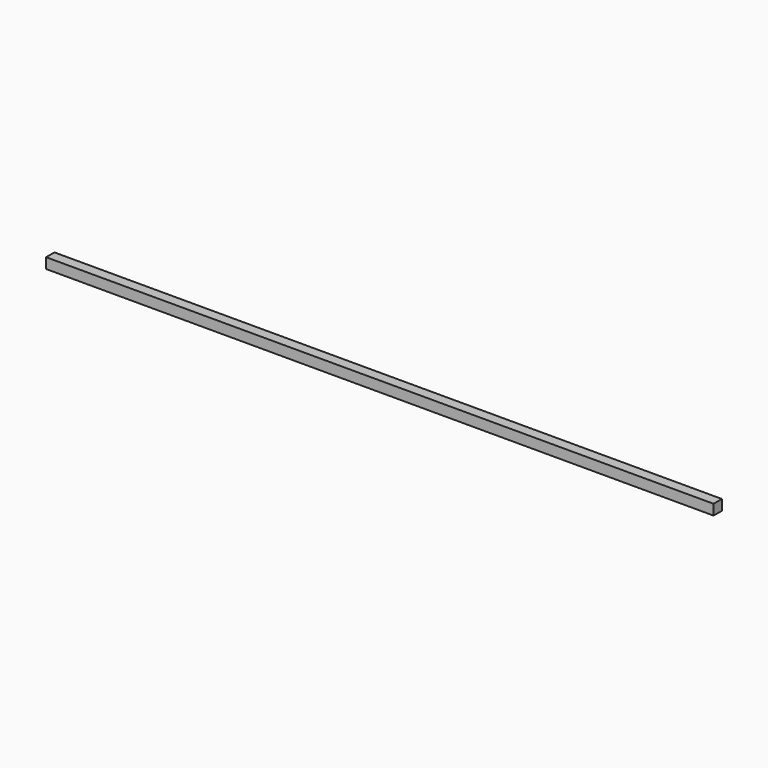
from build123d import *

# Parameters (mm, degrees)
F0_W     = 203.2
F0_H     = 3.175
F1_DEPTH = 3.175


# Not quite as in the source:
# - a length typed as a fraction of an inch, garbled in the dataset ("3 / 203.2 mm" for 3/8 in), is restored


with BuildPart() as f1:
    # F0 (on Front) → F1 (new body)
    with BuildSketch(Plane.XZ):
        with Locations((-3.4536693711, -8.6084658129)):
            Rectangle(F0_W, F0_H)
    extrude(amount=F1_DEPTH)


solid = f1.part
